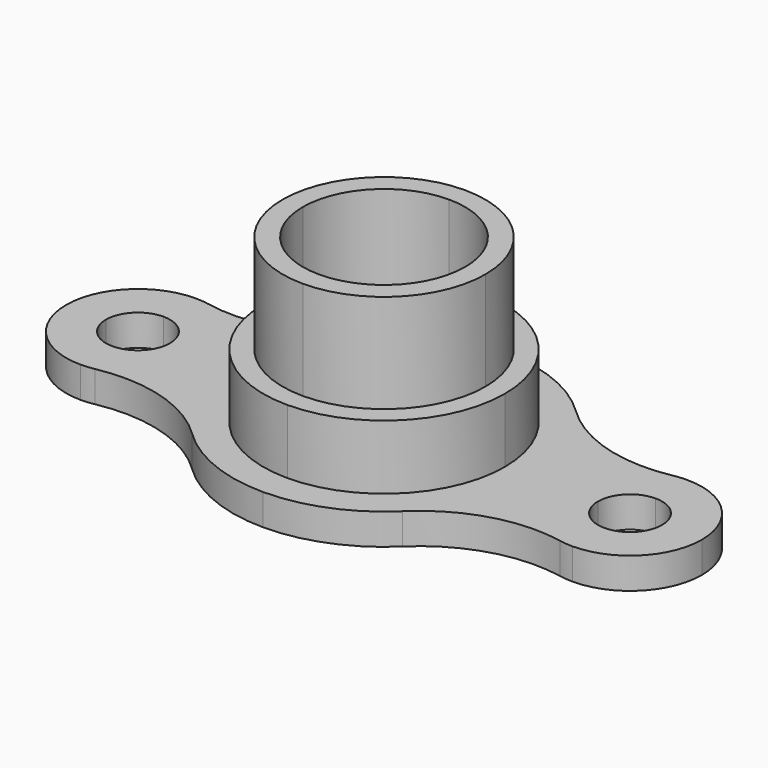
from build123d import *

# Parameters (mm, degrees)
F1_DEPTH = 1.397
F2_DEPTH = 8.7376
F3_DEPTH = 4.2926


# Not quite as in the source:
# - ends of sketch curves that miss each other by under 0.0002 mm in the source are joined


with BuildPart() as f1:
    # F0 (on Top) → F1 (new body)
    with BuildSketch(Plane.XY):
        with BuildLine():
            ThreePointArc((-5.4345187307, 0), (-3.8427850469, 3.8427850469), (0, 5.4345187307))
            Line((0, 5.4345187307), (0, 6.7959154799))
            ThreePointArc((0, 6.7959154799), (-2.5520653679, 6.2985259837), (-4.7305620794, 4.8791648489))
            ThreePointArc((-4.7305620794, 4.8791648489), (-7.3841557332, 3.3252325154), (-10.4555039298, 3.1733212198))
            ThreePointArc((-10.4555039298, 3.1733212198), (-10.7604870325, 3.2172453575), (-11.0682662539, 3.2319337461))
            Line((-11.0682662539, 3.2319337461), (-11.0682662539, 1.438874613))
            ThreePointArc((-11.0682662539, 1.438874613), (-10.0508282577, 1.0174379961), (-9.6293916409, 0))
            Line((-9.6293916409, 0), (-5.4345187307, 0))
        make_face()
        with BuildLine():
            ThreePointArc((-12.5071408669, 0), (-12.08570425, 1.0174379961), (-11.0682662539, 1.438874613))
            Line((-11.0682662539, 1.438874613), (-11.0682662539, 3.2319337461))
            ThreePointArc((-11.0682662539, 3.2319337461), (-13.3535885221, 2.2853222682), (-14.3002, 0))
            Line((-14.3002, 0), (-12.5071408669, 0))
        make_face()
        with BuildLine():
            Line((-11.0682662539, -3.2319337461), (-11.0682662539, -1.438874613))
            ThreePointArc((-11.0682662539, -1.438874613), (-12.08570425, -1.0174379961), (-12.5071408669, 0))
            Line((-12.5071408669, 0), (-14.3002, 0))
            ThreePointArc((-14.3002, 0), (-13.3535885221, -2.2853222682), (-11.0682662539, -3.2319337461))
        make_face()
        with BuildLine():
            Line((0, -6.7959154799), (0, -5.4345187307))
            ThreePointArc((0, -5.4345187307), (-3.8427850469, -3.8427850469), (-5.4345187307, 0))
            Line((-5.4345187307, 0), (-9.6293916409, 0))
            ThreePointArc((-9.6293916409, 0), (-10.0508282577, -1.0174379961), (-11.0682662539, -1.438874613))
            Line((-11.0682662539, -1.438874613), (-11.0682662539, -3.2319337461))
            ThreePointArc((-11.0682662539, -3.2319337461), (-10.7604870325, -3.2172453575), (-10.4555053814, -3.1733137022))
            ThreePointArc((-10.4555053814, -3.1733137022), (-7.3841557332, -3.3252325154), (-4.7305659764, -4.8791688684))
            ThreePointArc((-4.7305659764, -4.8791688684), (-2.5520653679, -6.2985259837), (0, -6.7959154799))
        make_face()
        with BuildLine():
            ThreePointArc((0, -5.4345187307), (3.8427850469, -3.8427850469), (5.4345187307, 0))
            Line((5.4345187307, 0), (4.5601256966, 0))
            ThreePointArc((4.5601256966, 0), (3.2244958031, -3.2244958031), (0, -4.5601256966))
            Line((0, -4.5601256966), (0, -5.4345187307))
        make_face()
        with BuildLine():
            ThreePointArc((-5.4345187307, 0), (-3.8427850469, -3.8427850469), (0, -5.4345187307))
            Line((0, -5.4345187307), (0, -4.5601256966))
            ThreePointArc((0, -4.5601256966), (-3.2244958031, -3.2244958031), (-4.5601256966, 0))
            Line((-4.5601256966, 0), (-5.4345187307, 0))
        make_face()
        with BuildLine():
            Line((0, 4.5601256966), (0, 5.4345187307))
            ThreePointArc((0, 5.4345187307), (-3.8427850469, 3.8427850469), (-5.4345187307, 0))
            Line((-5.4345187307, 0), (-4.5601256966, 0))
            ThreePointArc((-4.5601256966, 0), (-3.2244958031, 3.2244958031), (0, 4.5601256966))
        make_face()
        with BuildLine():
            Line((4.5601256966, 0), (5.4345187307, 0))
            ThreePointArc((5.4345187307, 0), (3.8427850469, 3.8427850469), (0, 5.4345187307))
            Line((0, 5.4345187307), (0, 4.5601256966))
            ThreePointArc((0, 4.5601256966), (3.2244958031, 3.2244958031), (4.5601256966, 0))
        make_face()
        with BuildLine():
            ThreePointArc((0, 5.4345187307), (3.8427850469, 3.8427850469), (5.4345187307, 0))
            Line((5.4345187307, 0), (9.6293916409, 0))
            ThreePointArc((9.6293916409, 0), (10.0508282577, 1.0174379961), (11.0682662539, 1.438874613))
            Line((11.0682662539, 1.438874613), (11.0682662539, 3.2319337461))
            ThreePointArc((11.0682662539, 3.2319337461), (10.7604870325, 3.2172453575), (10.4555053814, 3.1733137022))
            ThreePointArc((10.4555053814, 3.1733137022), (7.3841557332, 3.3252325154), (4.7305659764, 4.8791688684))
            ThreePointArc((4.7305659764, 4.8791688684), (2.5520653679, 6.2985259837), (0, 6.7959154799))
            Line((0, 6.7959154799), (0, 5.4345187307))
        make_face()
        with BuildLine():
            Line((9.6293916409, 0), (5.4345187307, 0))
            ThreePointArc((5.4345187307, 0), (3.8427850469, -3.8427850469), (0, -5.4345187307))
            Line((0, -5.4345187307), (0, -6.7959154799))
            ThreePointArc((0, -6.7959154799), (2.5520653679, -6.2985259837), (4.7305620794, -4.8791648489))
            ThreePointArc((4.7305620794, -4.8791648489), (7.3841557332, -3.3252325154), (10.4555039298, -3.1733212198))
            ThreePointArc((10.4555039298, -3.1733212198), (10.7604870325, -3.2172453575), (11.0682662539, -3.2319337461))
            Line((11.0682662539, -3.2319337461), (11.0682662539, -1.438874613))
            ThreePointArc((11.0682662539, -1.438874613), (10.0508282577, -1.0174379961), (9.6293916409, 0))
        make_face()
        with BuildLine():
            ThreePointArc((12.5071408669, 0), (12.08570425, -1.0174379961), (11.0682662539, -1.438874613))
            Line((11.0682662539, -1.438874613), (11.0682662539, -3.2319337461))
            ThreePointArc((11.0682662539, -3.2319337461), (13.3535885221, -2.2853222682), (14.3002, 0))
            Line((14.3002, 0), (12.5071408669, 0))
        make_face()
        with BuildLine():
            Line((11.0682662539, 3.2319337461), (11.0682662539, 1.438874613))
            ThreePointArc((11.0682662539, 1.438874613), (12.08570425, 1.0174379961), (12.5071408669, 0))
            Line((12.5071408669, 0), (14.3002, 0))
            ThreePointArc((14.3002, 0), (13.3535885221, 2.2853222682), (11.0682662539, 3.2319337461))
        make_face()
    extrude(amount=F1_DEPTH)

    # F0 (on Top) → F2 (join)
    with BuildSketch(Plane.XY):
        with BuildLine():
            Line((0, 3.6514210372), (0, 4.5601256966))
            ThreePointArc((0, 4.5601256966), (-3.2244958031, 3.2244958031), (-4.5601256966, 0))
            Line((-4.5601256966, 0), (-3.6514210372, 0))
            ThreePointArc((-3.6514210372, 0), (-2.5819445763, 2.5819445763), (0, 3.6514210372))
        make_face()
        with BuildLine():
            Line((3.6514210372, 0), (4.5601256966, 0))
            ThreePointArc((4.5601256966, 0), (3.2244958031, 3.2244958031), (0, 4.5601256966))
            Line((0, 4.5601256966), (0, 3.6514210372))
            ThreePointArc((0, 3.6514210372), (2.5819445763, 2.5819445763), (3.6514210372, 0))
        make_face()
        with BuildLine():
            ThreePointArc((0, -4.5601256966), (3.2244958031, -3.2244958031), (4.5601256966, 0))
            Line((4.5601256966, 0), (3.6514210372, 0))
            ThreePointArc((3.6514210372, 0), (2.5819445763, -2.5819445763), (0, -3.6514210372))
            Line((0, -3.6514210372), (0, -4.5601256966))
        make_face()
        with BuildLine():
            ThreePointArc((-4.5601256966, 0), (-3.2244958031, -3.2244958031), (0, -4.5601256966))
            Line((0, -4.5601256966), (0, -3.6514210372))
            ThreePointArc((0, -3.6514210372), (-2.5819445763, -2.5819445763), (-3.6514210372, 0))
            Line((-3.6514210372, 0), (-4.5601256966, 0))
        make_face()
    extrude(amount=F2_DEPTH)

    # F0 (on Top) → F3 (join)
    with BuildSketch(Plane.XY):
        with BuildLine():
            ThreePointArc((-5.4345187307, 0), (-3.8427850469, -3.8427850469), (0, -5.4345187307))
            Line((0, -5.4345187307), (0, -4.5601256966))
            ThreePointArc((0, -4.5601256966), (-3.2244958031, -3.2244958031), (-4.5601256966, 0))
            Line((-4.5601256966, 0), (-5.4345187307, 0))
        make_face()
        with BuildLine():
            ThreePointArc((0, -5.4345187307), (3.8427850469, -3.8427850469), (5.4345187307, 0))
            Line((5.4345187307, 0), (4.5601256966, 0))
            ThreePointArc((4.5601256966, 0), (3.2244958031, -3.2244958031), (0, -4.5601256966))
            Line((0, -4.5601256966), (0, -5.4345187307))
        make_face()
        with BuildLine():
            Line((4.5601256966, 0), (5.4345187307, 0))
            ThreePointArc((5.4345187307, 0), (3.8427850469, 3.8427850469), (0, 5.4345187307))
            Line((0, 5.4345187307), (0, 4.5601256966))
            ThreePointArc((0, 4.5601256966), (3.2244958031, 3.2244958031), (4.5601256966, 0))
        make_face()
        with BuildLine():
            Line((0, 4.5601256966), (0, 5.4345187307))
            ThreePointArc((0, 5.4345187307), (-3.8427850469, 3.8427850469), (-5.4345187307, 0))
            Line((-5.4345187307, 0), (-4.5601256966, 0))
            ThreePointArc((-4.5601256966, 0), (-3.2244958031, 3.2244958031), (0, 4.5601256966))
        make_face()
    extrude(amount=F3_DEPTH)


solid = f1.part
